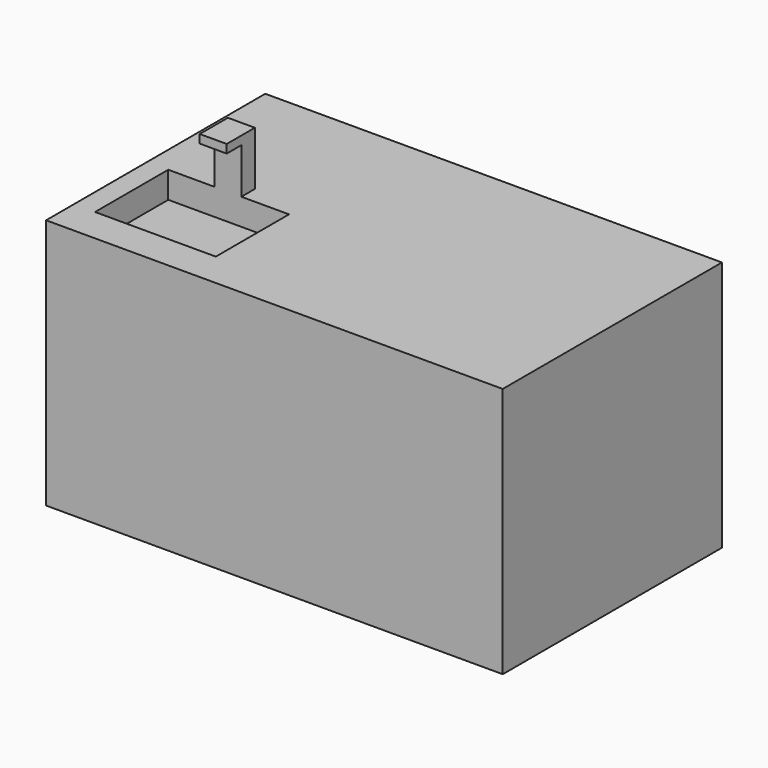
from build123d import *

# Parameters (mm, degrees)
F0_W     = 1524
F0_H     = 914.4
F1_DEPTH = 838.2
F2_W     = 403.0548334122
F2_H     = 305.4204545915
F3_DEPTH = 88.392
F4_W     = 90.1145935059
F4_H     = 56.3738569617
F5_DEPTH = 179.832
F6_W     = 90.1145935059
F6_H     = 28.3284043617
F7_DEPTH = 60.96


with BuildPart() as f1:
    # F0 (on Top) → F1 (new body)
    with BuildSketch(Plane.XY):
        with Locations((-449.5147587423, 11.9446208701)):
            Rectangle(F0_W, F0_H)
    extrude(amount=F1_DEPTH)

    # F2 (on face) → F3 (cut)
    with BuildSketch(Plane.XY.offset(838.2)):
        with Locations((-939.5418763161, -176.386596635)):
            Rectangle(F2_W, F2_H)
    extrude(amount=-F3_DEPTH, mode=Mode.SUBTRACT)

    # F4 (on face) → F5 (join)
    with BuildSketch(Plane.XY.offset(838.2)):
        with Locations((-942.1632885933, 4.5105591416)):
            Rectangle(F4_W, F4_H)
    extrude(amount=F5_DEPTH)

    # F6 (on face) → F7 (join)
    with BuildSketch(Plane.XZ.offset(23.6763693392)):
        with Locations((-942.1632885933, 1003.8677978191)):
            Rectangle(F6_W, F6_H)
    extrude(amount=F7_DEPTH)


solid = f1.part
